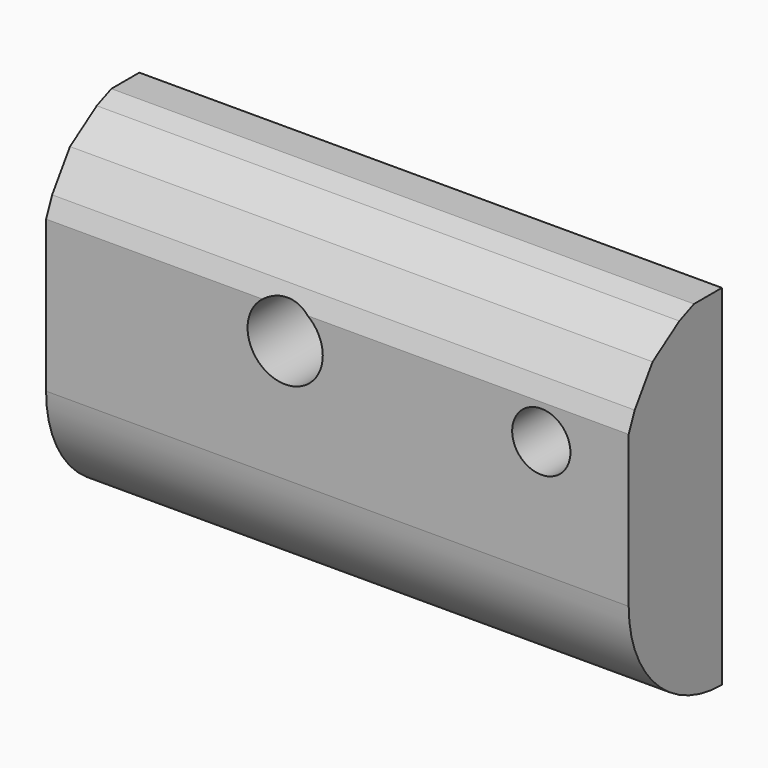
from build123d import *

# Parameters (mm, degrees)
F0_W        = 127
F0_H        = 76.2
F0_R        = 6.35
F1_DEPTH    = 25.4
F2_R        = 8.1972505448
F3_DEPTH    = 19.812
F4_SIZE     = 12.7
F5_SIZE     = 5.08
F6_T1_DEPTH = 153.3415311919
F7_SIZE     = 5.08
F8_T1_DEPTH = 153.3972220228
F9_R        = 25.39999


# Not quite as in the source:
# - a fillet or chamfer that OpenCascade refuses, or shapes differently, is made with other operations: its cross-section is extruded or revolved along the edge and cut away or added
# - a fillet or chamfer is up to 0.001 mm smaller than in the source, because OpenCascade refuses the exact size


with BuildPart() as f1:
    # F0 (on Front) → F1 (new body)
    with BuildSketch(Plane.XZ):
        with Locations((30.7051779926, 16.4221930265)):
            Rectangle(F0_W, F0_H)
        with Locations((75.1551779926, 29.1221930265)):
            Circle(F0_R, mode=Mode.SUBTRACT)
    extrude(amount=F1_DEPTH)

    # F2 (on face) → F3 (cut)
    with BuildSketch(Plane.XZ.offset(25.4)):
        with Locations((19.3208176643, 30.1677044481)):
            Circle(F2_R)
    extrude(amount=-F3_DEPTH, mode=Mode.SUBTRACT)

    # F4
    f4_edges = [f1.edges().sort_by_distance(p)[0] for p in [
        (30.705178, -25.4, 54.522193),
    ]]
    chamfer(f4_edges, length=F4_SIZE)

    # F5
    f5_edges = [f1.edges().sort_by_distance(p)[0] for p in [
        (30.705178, -12.7, 54.522193),
    ]]
    chamfer(f5_edges, length=F5_SIZE)

    # F6: chamfer of 5.08 on 1 edges, made by hand

    # F6_s2 → F6_t1 (cut)
    with BuildSketch(Plane.YZ.offset(-45.9655876034)):
        Polygon((-21.8078975516, 45.414295475), (-25.4, 36.7421930265), (-25.4, 41.8221930265), align=None)
    extrude(amount=F6_T1_DEPTH, mode=Mode.SUBTRACT)

    # F7
    f7_edges = [f1.edges().sort_by_distance(p)[0] for p in [
        (30.705178, -21.807898, 45.414295),
    ]]
    chamfer(f7_edges, length=F7_SIZE)

    # F8: chamfer of 5.08 on 1 edges, made by hand

    # F8_s2 → F8_t1 (cut)
    with BuildSketch(Plane.YZ.offset(-45.9934330188)):
        Polygon((-19.8842048969, 47.3379881297), (-11.5987944233, 52.8741224145), (-16.2921024484, 50.9300905781), align=None)
    extrude(amount=F8_T1_DEPTH, mode=Mode.SUBTRACT)

    # F9 (radius 25.4 in the source; OpenCascade refuses exactly that, so slightly less here)
    f9_edges = [f1.edges().sort_by_distance(p)[0] for p in [
        (30.705178, -25.4, -21.677807),
    ]]
    fillet(f9_edges, radius=F9_R)


solid = f1.part
